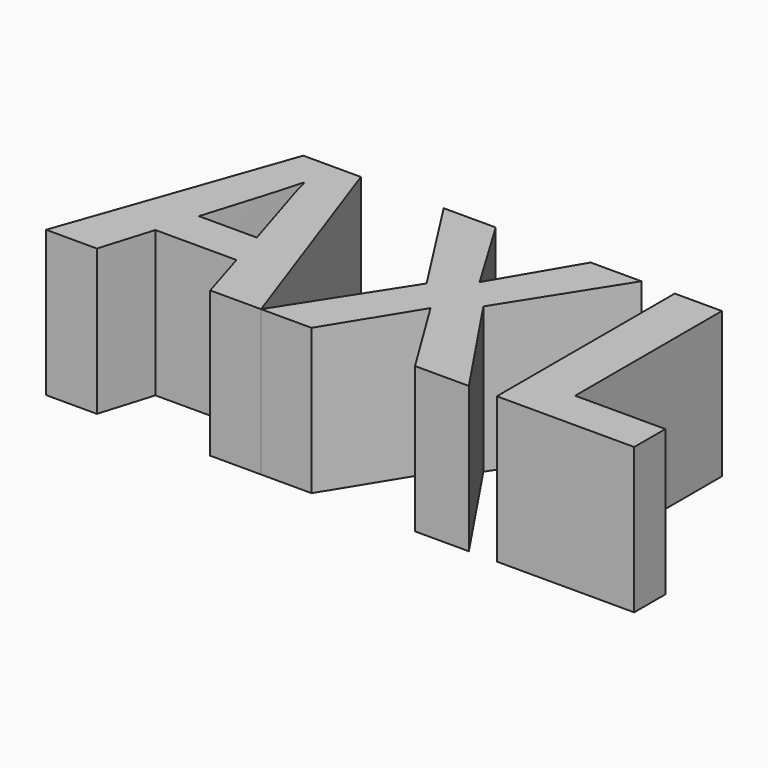
from build123d import *

# Parameters (mm, degrees)
F0_TEXT_SIZE = 54.3548363364
F1_DEPTH     = 25.4


# Not quite as in the source:
# - Text() gives the source's letters only with a copy of the font that has no kerning and outlines rounded to 1/6400 em; it was checked with that copy


with BuildPart() as f1:
    # F0 (on Top) → F1 (new body)
    with BuildSketch(Plane.XY):
        with Locations((-63.9717951417, 0)):
            Text('AXL', F0_TEXT_SIZE, font='Open Sans', font_style=FontStyle.BOLD, text_align=(TextAlign.LEFT, TextAlign.BOTTOM))
    extrude(amount=F1_DEPTH)


solid = f1.part
